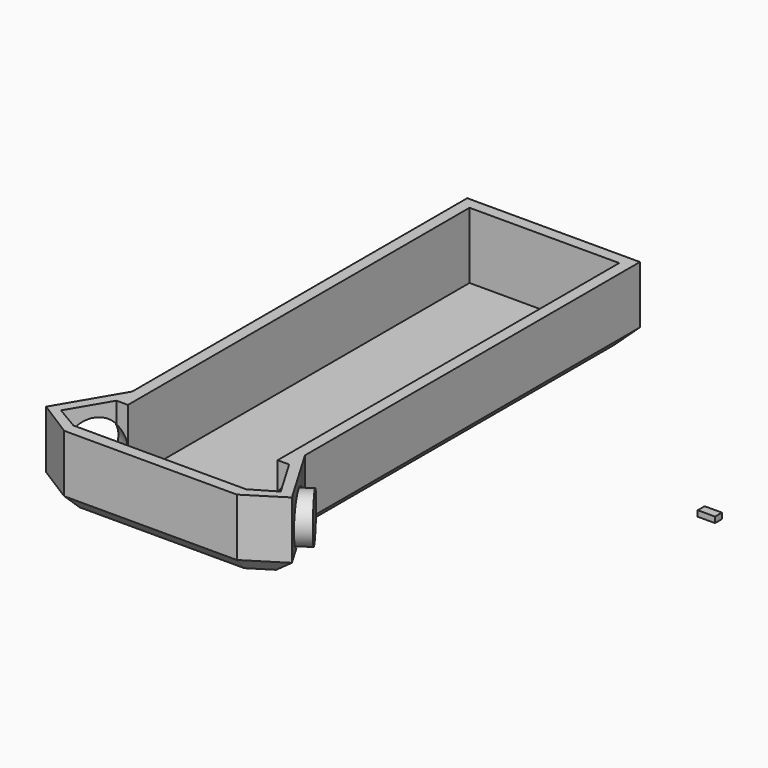
from build123d import *

# Parameters (mm, degrees)
F1_DEPTH      = 25
F0_W          = 4
F0_H          = 18.6791904594
F2_DEPTH      = 2
F4_DEPTH      = 8
F5_DEPTH      = 10
F6_SIZE       = 1
F0_W_2        = 6
F0_H_2        = 3
F7_DEPTH      = 2
F11_ANGLE     = 90
F14_ANGLE     = -35.3879511654
F17_DEPTH     = 8
F18_T1_DEPTH  = 85.7168298797
F18_T3_DEPTH  = 40.7217896719
F18_T5_DEPTH  = 40.7217896719
F18_T10_DEPTH = 50.7168298797
F18_T15_DEPTH = 171.1796252878
F18_T20_DEPTH = 171.1796252878
F18_T25_DEPTH = 50.7168298797
F18_T31_DEPTH = 171.1796252878
F18_T35_DEPTH = 50.7168298797
F18_T42_DEPTH = 171.1796252878
F18_T46_DEPTH = 50.7168298797


# Not quite as in the source:
# - a fillet or chamfer that OpenCascade refuses, or shapes differently, is made with other operations: its cross-section is extruded or revolved along the edge and cut away or added


with BuildPart() as f1:
    # F0 (on Top) → F1 (new body)
    with BuildSketch(Plane.XY):
        Polygon((-60, -49.5964816809), (-60, -53.5964816809), (0, -53.5964816809), (0, -49.5964816809), (-4, -49.5964816809), (-56, -49.5964816809), align=None)
        Polygon((-72.6944404511, -45.5964816809), (-60, -53.5964816809), (-60, -49.5964816809), (-68.171107597, -44.7802745279), (-71.171107597, -43.0120171298), align=None)
        Polygon((-63, -29.1490338234), (-60, -30.9172912215), (-60, -24.059277089), align=None)
        Polygon((-63, -29.1490338234), (-71.171107597, -43.0120171298), (-68.171107597, -44.7802745279), (-60, -30.9172912215), align=None)
        Polygon((-60, -24.059277089), (-60, -30.9172912215), (-56, -30.9172912215), (-56, 117.4035183191), (-4, 117.4035183191), (-4, -30.9172912215), (0, -30.9172912215), (0, -24.059277089), (0, 121.4035183191), (-60, 121.4035183191), align=None)
        Polygon((0, -24.059277089), (0, -30.9172912215), (3, -29.1490338234), align=None)
        Polygon((8.171107597, -44.7802745279), (11.171107597, -43.0120171298), (3, -29.1490338234), (0, -30.9172912215), align=None)
        Polygon((0, -49.5964816809), (0, -53.5964816809), (12.6944404511, -45.5964816809), (11.171107597, -43.0120171298), (8.171107597, -44.7802745279), align=None)
    extrude(amount=F1_DEPTH)

    # F0 (on Top) → F2 (join)
    with BuildSketch(Plane.XY):
        Polygon((-56, -30.9172912215), (-56, -49.5964816809), (-4, -49.5964816809), (-4, -30.9172912215), (-4, 117.4035183191), (-56, 117.4035183191), align=None)
        Polygon((0, -30.9172912215), (0, -49.5964816809), (8.171107597, -44.7802745279), align=None)
        with Locations((-2, -40.2568864512)):
            Rectangle(F0_W, F0_H)
        Polygon((-68.171107597, -44.7802745279), (-60, -49.5964816809), (-60, -30.9172912215), align=None)
        with Locations((-58, -40.2568864512)):
            Rectangle(F0_W, F0_H)
    extrude(amount=F2_DEPTH)

    # F3 (on face) → F4 (cut)
    with BuildSketch(Plane(origin=(-10.5245964608, -6.2033985179, 0), x_dir=(-0.507777618, 0.8614881837, 0), z_dir=(0.8614881837, 0.507777618, 0))):
        with BuildLine():
            ThreePointArc((-33.2267829199, 4), (-27.2163752798, 6.4895923599), (-24.7267829199, 12.5))
            ThreePointArc((-24.7267829199, 12.5), (-27.2163752798, 18.5104076401), (-33.2267829199, 21))
            Line((-33.2267829199, 21), (-33.2267829199, 4))
        make_face()
        with BuildLine():
            Line((-33.2267829199, 4), (-33.2267829199, 21))
            ThreePointArc((-33.2267829199, 21), (-41.7267829199, 12.5), (-33.2267829199, 4))
        make_face()
    extrude(amount=-F4_DEPTH, mode=Mode.SUBTRACT)

    # F16 (on face) → F17 (cut)
    with BuildSketch(Plane(origin=(-34.0051169759, 20.043266555, 0), x_dir=(-0.507777618, -0.8614881837, 0), z_dir=(-0.8614881837, 0.507777618, 0))):
        with BuildLine():
            Line((69.7038476428, 6.4895923599), (57.6830323626, 18.5104076401))
            ThreePointArc((57.6830323626, 18.5104076401), (57.6830323626, 6.4895923599), (69.7038476428, 6.4895923599))
        make_face()
        with BuildLine():
            ThreePointArc((72.1934400027, 12.5), (66.9462491778, 20.3529760263), (57.6830323626, 18.5104076401))
            Line((57.6830323626, 18.5104076401), (69.7038476428, 6.4895923599))
            ThreePointArc((69.7038476428, 6.4895923599), (71.546416029, 9.2471908249), (72.1934400027, 12.5))
        make_face()
    extrude(amount=-F17_DEPTH, mode=Mode.SUBTRACT)

    # F18: chamfer of 5 on 8 edges, made by hand

    # F18_s2 → F18_t1 (cut)
    with BuildSketch(Plane.YZ.offset(-72.8584149398)):
        Polygon((-53.5964816809, 5), (-48.5964816809, 0), (-53.5964816809, 0), align=None)
        Polygon((121.4035183191, 5), (116.4035183191, 0), (121.4035183191, 0), align=None)
    extrude(amount=F18_T1_DEPTH, mode=Mode.SUBTRACT)

    # F18_s4 → F18_t3 (cut)
    with BuildSketch(Plane(origin=(-42.3422783558, 26.6839825001, 0), x_dir=(0, 0, 1), z_dir=(0.8460162924, -0.5331570435, 0))):
        Polygon((5, 77.3329193249), (0, 72.3329193249), (0, 77.3329193249), align=None)
    extrude(amount=F18_T3_DEPTH, mode=Mode.SUBTRACT)

    # F18_s6 → F18_t5 (cut)
    with BuildSketch(Plane(origin=(-35.0536331835, -22.090699196, 0), x_dir=(0, 0, 1), z_dir=(0.8460162924, 0.5331570435, 0))):
        Polygon((5, 45.3434967176), (0, 40.3434967176), (0, 45.3434967176), align=None)
    extrude(amount=F18_T5_DEPTH, mode=Mode.SUBTRACT)


with BuildPart() as f5:
    # F0 (on Top) → F5 (new body)
    with BuildSketch(Plane.XY):
        with BuildLine():
            ThreePointArc((122.4339852025, 55.2492514253), (130.4339852025, 47.2492514253), (138.4339852025, 55.2492514253))
            Line((138.4339852025, 55.2492514253), (122.4339852025, 55.2492514253))
        make_face()
        with BuildLine():
            Line((122.4339852025, 55.2492514253), (138.4339852025, 55.2492514253))
            ThreePointArc((138.4339852025, 55.2492514253), (130.4339852025, 63.2492514253), (122.4339852025, 55.2492514253))
        make_face()
    extrude(amount=F5_DEPTH)

    # F6
    f6_edges = [f5.edges().sort_by_distance(p)[0] for p in [
        (122.433985, 55.249251, 10),
    ]]
    chamfer(f6_edges, length=F6_SIZE)


with BuildPart() as f7:
    # F0 (on Top) → F7 (new body)
    with BuildSketch(Plane.XY):
        with Locations((78.7412314415, 53.3295951188)):
            Rectangle(F0_W_2, F0_H_2)
    extrude(amount=F7_DEPTH)


with BuildPart() as f5_1:
    # F8: moved
    add(f5.part.moved(Location((-115.6432256103, -84.226578474, 0))))


with BuildPart() as f5_2:
    # F11: moved
    add(f5_1.part.rotate(Axis((13.3097898215, -28.9531024173, 4), (0, -1, 0)), F11_ANGLE))


with BuildPart() as f5_3:
    # F14: moved
    add(f5_2.part.rotate(Axis((13.3097898215, -29.0680099279, 5.3557939827), (0, 0, -1)), F14_ANGLE))


with BuildPart() as f5_4:
    # F15: moved
    add(f5_3.part.moved(Location((-6.7074596882, -5.5138133466, 7.0042535663))))


with BuildPart() as f18_tool8:
    # F18_s9 → F18_t10 (new body)
    with BuildSketch(Plane(origin=(29.748252222, -50.4704556945, 0), x_dir=(0, 0, 1), z_dir=(-0.507777618, 0.8614881837, 0))):
        Polygon((5, -12.2167624121), (0, -17.2167624121), (0, -12.2167624121), align=None)
    extrude(amount=F18_T10_DEPTH)

    split(bisect_by=Plane.YZ, keep=Keep.TOP)


with BuildPart() as f1_1:
    add(f1.part)

    # F18_t7: cut F18_tool8
    add(f18_tool8.part, mode=Mode.SUBTRACT)


with BuildPart() as f18_tool13:
    # F18_s14 → F18_t15 (new body)
    with BuildSketch(Plane.XZ.offset(36.9176920288)):
        Polygon((0, 5), (-5, 0), (0, 0), align=None)
    extrude(amount=-F18_T15_DEPTH)

    split(bisect_by=Plane(origin=(-10.5245964608, -6.2033985179, 0), x_dir=(0, 0, 1), z_dir=(0.8614881837, 0.507777618, 0)), keep=Keep.TOP)


with BuildPart() as f1_2:
    add(f1_1.part)

    # F18_t12: cut F18_tool13
    add(f18_tool13.part, mode=Mode.SUBTRACT)


with BuildPart() as f18_tool18:
    # F18_s19 → F18_t20 (new body)
    with BuildSketch(Plane.XZ.offset(-134.261933259)):
        Polygon((-60, 5), (-55, 0), (-60, 0), align=None)
    extrude(amount=F18_T20_DEPTH)

    split(bisect_by=Plane(origin=(-34.0051169759, 20.043266555, 0), x_dir=(0, 0, 1), z_dir=(-0.8614881837, 0.507777618, 0)), keep=Keep.TOP)


with BuildPart() as f1_3:
    add(f1_2.part)

    # F18_t17: cut F18_tool18
    add(f18_tool18.part, mode=Mode.SUBTRACT)


with BuildPart() as f18_tool23:
    # F18_s24 → F18_t25 (new body)
    with BuildSketch(Plane(origin=(-19.4656677141, -33.0251711125, 0), x_dir=(0, 0, 1), z_dir=(-0.507777618, -0.8614881837, 0))):
        Polygon((5, 39.4725286084), (0, 34.4725286084), (0, 39.4725286084), align=None)
    extrude(amount=F18_T25_DEPTH)

    split(bisect_by=Plane.YZ.offset(-60), keep=Keep.BOTTOM)


with BuildPart() as f1_4:
    add(f1_3.part)

    # F18_t22: cut F18_tool23
    add(f18_tool23.part, mode=Mode.SUBTRACT)


with BuildPart() as f18_tool29:
    # F18_s30 → F18_t31 (new body)
    with BuildSketch(Plane.XZ.offset(36.9176920288)):
        Polygon((0, 5), (-5, 0), (0, 0), align=None)
    extrude(amount=-F18_T31_DEPTH)

    split(bisect_by=Plane(origin=(-10.5245964608, -6.2033985179, 0), x_dir=(0, 0, 1), z_dir=(-0.8614881837, -0.507777618, 0)), keep=Keep.TOP)


with BuildPart() as f18_tool33:
    # F18_s34 → F18_t35 (new body)
    with BuildSketch(Plane(origin=(29.748252222, -50.4704556945, 0), x_dir=(0, 0, 1), z_dir=(-0.507777618, 0.8614881837, 0))):
        Polygon((5, -12.2167624121), (0, -17.2167624121), (0, -12.2167624121), align=None)
    extrude(amount=F18_T35_DEPTH)

    split(bisect_by=Plane.YZ, keep=Keep.BOTTOM)


with BuildPart() as f18_tool29_1:
    add(f18_tool29.part)

    # F18_t37: intersect F18_tool33
    add(f18_tool33.part, mode=Mode.INTERSECT)


with BuildPart() as f1_5:
    add(f1_4.part)

    # F18_t27: cut F18_tool29
    add(f18_tool29_1.part, mode=Mode.SUBTRACT)


with BuildPart() as f18_tool40:
    # F18_s41 → F18_t42 (new body)
    with BuildSketch(Plane.XZ.offset(-134.261933259)):
        Polygon((-60, 5), (-55, 0), (-60, 0), align=None)
    extrude(amount=F18_T42_DEPTH)

    split(bisect_by=Plane(origin=(-34.0051169759, 20.043266555, 0), x_dir=(0, 0, 1), z_dir=(0.8614881837, -0.507777618, 0)), keep=Keep.TOP)


with BuildPart() as f18_tool44:
    # F18_s45 → F18_t46 (new body)
    with BuildSketch(Plane(origin=(-19.4656677141, -33.0251711125, 0), x_dir=(0, 0, 1), z_dir=(-0.507777618, -0.8614881837, 0))):
        Polygon((5, 39.4725286084), (0, 34.4725286084), (0, 39.4725286084), align=None)
    extrude(amount=F18_T46_DEPTH)

    split(bisect_by=Plane.YZ.offset(-60), keep=Keep.TOP)


with BuildPart() as f18_tool40_1:
    add(f18_tool40.part)

    # F18_t48: intersect F18_tool44
    add(f18_tool44.part, mode=Mode.INTERSECT)


with BuildPart() as f1_6:
    add(f1_5.part)

    # F18_t38: cut F18_tool40
    add(f18_tool40_1.part, mode=Mode.SUBTRACT)


solid = Compound([f7.part, f5_4.part, f1_6.part])
